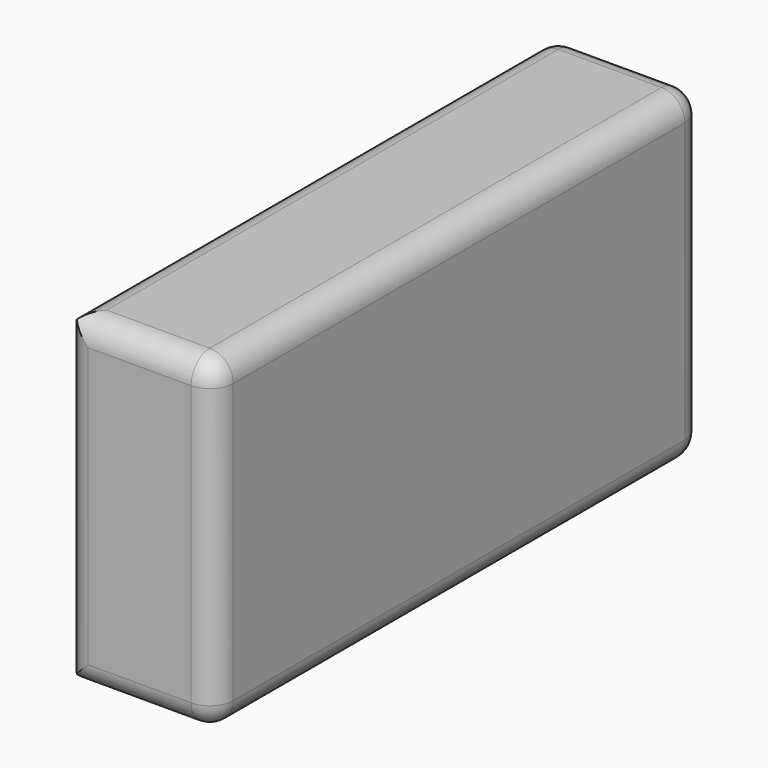
from build123d import *

# Parameters (mm, degrees)
F0_W        = 80.0341404974
F0_H        = 70.704229176
F1_DEPTH    = 132.588
F2_DEPTH    = 48.006
F3_DEPTH    = 47.498
F4_R        = 5.08
F5_T1_DEPTH = 85.944229176


# Not quite as in the source:
# - a fillet or chamfer that OpenCascade refuses, or shapes differently, is made with other operations: its cross-section is extruded or revolved along the edge and cut away or added


with BuildPart() as f1:
    # F0 (on Front) → F1 (new body)
    with BuildSketch(Plane.XZ):
        with Locations((-100.3818046302, 35.352114588)):
            Rectangle(F0_W, F0_H)
    extrude(amount=F1_DEPTH)

    # F2 (add): a face of the model
    f2_faces = [f1.faces().sort_by_distance(p)[0] for p in [
        (-60.3647343814, -66.294, 35.352114588),
    ]]
    extrude(f2_faces, amount=-F2_DEPTH)

    # F3 (cut): a face of the model
    f3_faces = [f1.faces().sort_by_distance(p)[0] for p in [
        (-60.3647343814, -66.294, 35.352114588),
    ]]
    extrude(f3_faces, amount=-F3_DEPTH, mode=Mode.SUBTRACT)

    # F4
    f4_edges = [f1.edges().sort_by_distance(p)[0] for p in [
        (-107.862734, -66.294, 70.704229),
        (-124.130805, -132.588, 70.704229),
        (-140.398875, -66.294, 70.704229),
        (-124.130805, 0, 70.704229),
        (-107.862734, -132.588, 35.352115),
        (-124.130805, -132.588, 0),
        (-107.862734, 0, 35.352115),
        (-107.862734, -66.294, 0),
        (-124.130805, 0, 0),
        (-140.398875, 0, 35.352115),
        (-140.398875, -66.294, 0),
    ]]
    fillet(f4_edges, radius=F4_R)

    # F5: fillet of radius 5.08 on 4 edges, made by hand

    # F5_s2 → F5_t1 (cut)
    with BuildSketch(Plane.XY.offset(-7.62)):
        with BuildLine():
            ThreePointArc((-135.3188748789, -132.588), (-138.9109773273, -131.1001024484), (-140.3988748789, -127.508))
            Line((-140.3988748789, -127.508), (-140.3988748789, -132.588))
            Line((-140.3988748789, -132.588), (-135.3188748789, -132.588))
        make_face()
    extrude(amount=F5_T1_DEPTH, mode=Mode.SUBTRACT)


solid = f1.part
